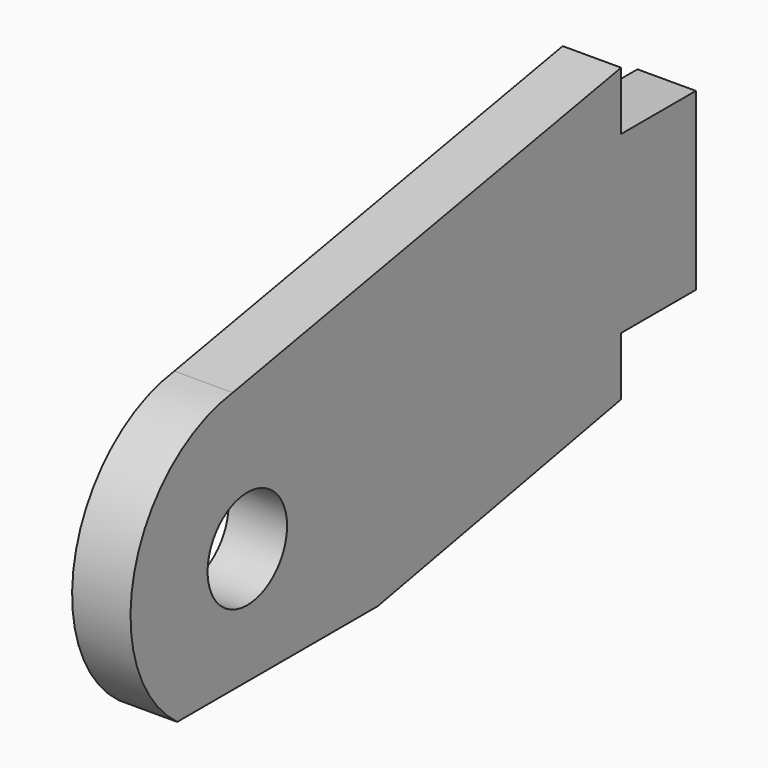
from build123d import *

# Parameters (mm, degrees)
F0_R     = 4.25
F0_W     = 8
F0_H     = 15
F1_DEPTH = 5


# Not quite as in the source:
# - a feature names something its author has since deleted; it is built from what else it names


with BuildPart() as f1:
    # F0 (on Right) → F1 (new body)
    with BuildSketch(Plane.YZ):
        with BuildLine():
            Line((-7.5, -10), (7.5, -10))
            ThreePointArc((7.5, -10), (11.5869510213, 4.689623229), (-1.5666059757, 12.4014412758))
            ThreePointArc((-1.5666059757, 12.4014412758), (-12.0833347544, 3.2004720296), (-7.5, -10))
        make_face()
        Circle(F0_R, mode=Mode.SUBTRACT)
        with BuildLine():
            ThreePointArc((-1.5666059757, 12.4014412758), (11.5869510213, 4.689623229), (7.5, -10))
            Line((7.5, -10), (13.9559781345, -10))
            Line((13.9559781345, -10), (40, -5))
            Line((40, -5), (40, 0))
            Line((40, 0), (40, 15))
            Line((40, 15), (40, 20))
            Line((40, 20), (-1.5666059757, 12.4014412758))
        make_face()
        with Locations((44, 7.5)):
            Rectangle(F0_W, F0_H)
    extrude(amount=F1_DEPTH)


solid = f1.part
